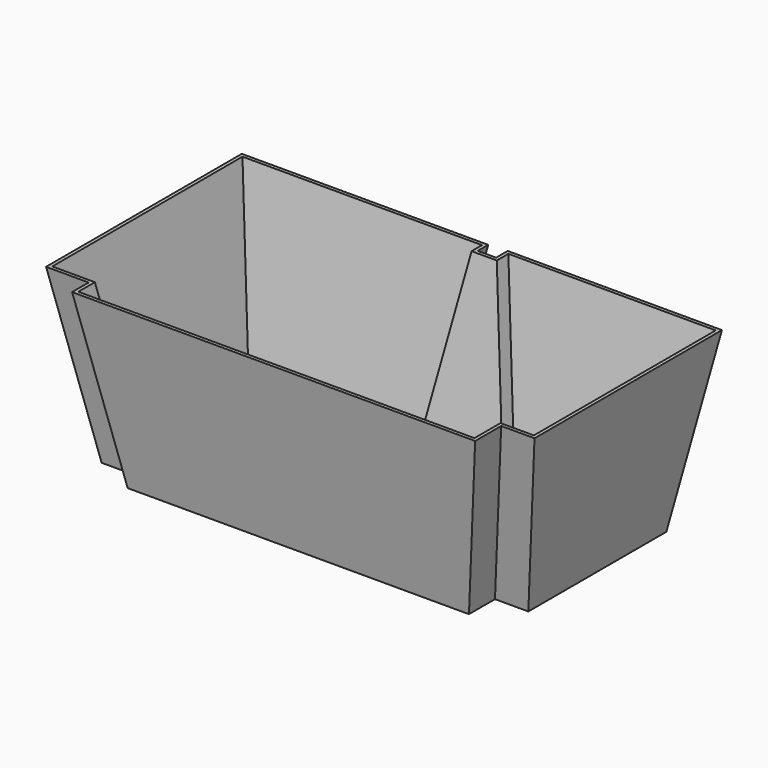
from build123d import *

# Parameters (mm, degrees)
F1_DEPTH               = 131.826
DRAFT_F1_DRAFTED_ANGLE = -10
F2_T                   = -2.54


# Not quite as in the source:
# - an extrude with a draft is written as a straight extrude whose walls are then drafted


with BuildPart() as f1:
    # F0 (on Top) → F1 (new body)
    with BuildSketch(Plane.XY):
        Polygon((20.9975820035, 76.288625598), (-39.307769388, 76.288625598), (-39.307769388, 86.107775569), (-178.3379018307, 86.107775569), (-178.3379018307, -51.6000725329), (-146.2680399418, -51.6000725329), (-146.2680399418, -67.208096385), (110.7110530138, -67.208096385), (110.7110530138, -42.7152328193), (135.8127295971, -42.7152328193), (135.8127295971, 87.1754735708), (20.9975820035, 87.1754735708), align=None)
    extrude(amount=F1_DEPTH)

    # draft_F1_drafted
    draft_f1_drafted_walls = [f1.faces().sort_by_distance(p)[0] for p in [
        (-9.1550936922, 76.288625598, 87.884),
        (-39.307769388, 81.1982005835, 87.884),
        (-108.8228356093, 86.107775569, 87.884),
        (-178.3379018307, 17.253851518, 87.884),
        (-162.3029708862, -51.6000725329, 87.884),
        (-146.2680399418, -59.4040844589, 87.884),
        (-17.778493464, -67.208096385, 87.884),
        (110.7110530138, -54.9616646022, 87.884),
        (123.2618913054, -42.7152328193, 87.884),
        (135.8127295971, 22.2301203758, 87.884),
        (78.4051558003, 87.1754735708, 87.884),
        (20.9975820035, 81.7320495844, 87.884),
    ]]
    draft(draft_f1_drafted_walls, neutral_plane=Plane.XY, angle=DRAFT_F1_DRAFTED_ANGLE)

    # F2
    f2_openings = [f1.faces().sort_by_distance(p)[0] for p in [
        (-21.338544, 10.920729, 131.826),
    ]]
    offset(amount=F2_T, openings=f2_openings, kind=Kind.INTERSECTION)


solid = f1.part
